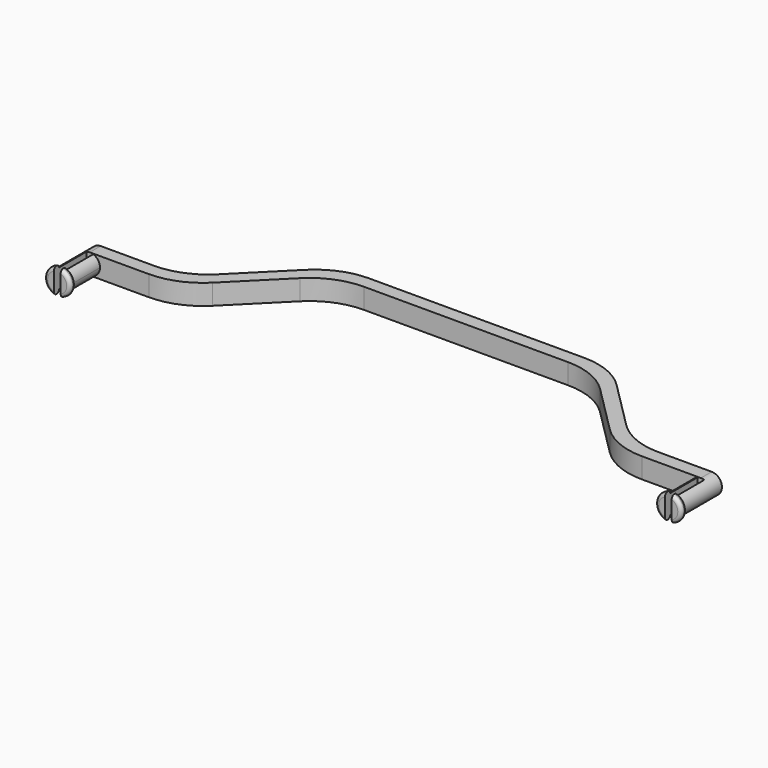
from build123d import *
from build123d import SkipClean  # not in build123d's __all__

# Parameters (mm, degrees)
F1_DEPTH  = 3
F2_R      = 10
F3_R      = 1.5
F4_DEPTH  = 2
F5_DEPTH  = 6
F6_R      = 1.9
F6_R_2    = 1.5
F7_DEPTH  = 1
F9_W      = 1
F9_H      = 10.6840910192
F9_W_2    = 7.2588436306
F9_H_2    = 0.5
F9_W_3    = 6.9682821631
F10_DEPTH = 6


# Not quite as in the source:
# - a fillet or chamfer that OpenCascade refuses, or shapes differently, is made with other operations: its cross-section is extruded or revolved along the edge and cut away or added
# - after a boolean that leaves OpenCascade's solid faulty, fix() repairs it


with BuildPart() as f1:
    # F0 (on Top) → F1 (new body)
    with BuildSketch(Plane.XY):
        Polygon((-45, 2), (-45, 0), (-32.1715728753, 0), (-33, 2), align=None)
        Polygon((-33, 2), (-32.1715728753, 0), (-19.1715728753, 13), (-20, 15), align=None)
        Polygon((-20, 15), (-19.1715728753, 13), (0, 13), (0, 15), align=None)
        Polygon((0, 15), (0, 13), (19.1715728753, 13), (20, 15), align=None)
        Polygon((20, 15), (19.1715728753, 13), (32.1715728753, 0), (33, 2), align=None)
        Polygon((33, 2), (32.1715728753, 0), (45, 0), (45, 2), align=None)
    extrude(amount=F1_DEPTH)

    # F2
    f2_edges = [f1.edges().sort_by_distance(p)[0] for p in [
        (-33, 2, 1.5),
        (-20, 15, 1.5),
        (20, 15, 1.5),
        (33, 2, 1.5),
        (32.171573, 0, 1.5),
        (19.171573, 13, 1.5),
        (-19.171573, 13, 1.5),
        (-32.171573, 0, 1.5),
    ]]
    fillet(f2_edges, radius=F2_R)

    # F3 (on face) → F4 (join, through all)
    with BuildSketch(Plane.XZ):
        with BuildLine():
            Line((-45, 0), (-45, 3))
            ThreePointArc((-45, 3), (-46.5, 1.5), (-45, 0))
        make_face()
        with Locations((45, 1.5)):
            Circle(F3_R)
    extrude(amount=-F4_DEPTH)

    # F3 (on face) → F5 (join)
    with BuildSketch(Plane.XZ):
        with BuildLine():
            Line((-45, 0), (-45, 3))
            ThreePointArc((-45, 3), (-46.5, 1.5), (-45, 0))
        make_face()
        with BuildLine():
            ThreePointArc((-45, 0), (-43.9393398282, 0.4393398282), (-43.5, 1.5))
            ThreePointArc((-43.5, 1.5), (-43.9393398282, 2.5606601718), (-45, 3))
            Line((-45, 3), (-45, 0))
        make_face()
        with Locations((45, 1.5)):
            Circle(F3_R)
    with SkipClean():  # cleaning this boolean's faces spoils the solid; the shape is the same uncleaned
        extrude(amount=F5_DEPTH)

    # F6 (on face) → F7 (join)
    with BuildSketch(Plane.XZ.offset(6)):
        with Locations((-45, 1.5)):
            Circle(F6_R)
        with Locations((-45, 1.5)):
            Circle(F6_R_2, mode=Mode.SUBTRACT)
        with Locations((45, 1.5)):
            Circle(F6_R)
    extrude(amount=-F7_DEPTH)

    add(f1.part.fix(), mode=Mode.REPLACE)

    # F8: fillet of radius 0.5 on 4 edges, made by hand

    # F8_s1 → F8_t2 (revolve, cut)
    with BuildSketch(Plane.XY.offset(1.5)):
        with BuildLine():
            ThreePointArc((-43.1, -5.5), (-43.2464466094, -5.8535533906), (-43.6, -6))
            Line((-43.6, -6), (-43.1, -6))
            Line((-43.1, -6), (-43.1, -5.5))
        make_face()
    revolve(axis=Axis((-45, -6, 1.5), (0, -1, 0)), mode=Mode.SUBTRACT)

    # F8_s3 → F8_t4 (revolve, cut)
    with BuildSketch(Plane.XY.offset(1.5)):
        with BuildLine():
            ThreePointArc((-43.5, -5), (-43.2127016654, -5.1736701825), (-43.1, -5.4898979486))
            Line((-43.1, -5.4898979486), (-43.1, -5))
            Line((-43.1, -5), (-43.5, -5))
        make_face()
    revolve(axis=Axis((-45, -5, 1.5), (0, -1, 0)), mode=Mode.SUBTRACT)

    # F8_s5 → F8_t6 (revolve, cut)
    with BuildSketch(Plane.XY.offset(1.5)):
        with BuildLine():
            ThreePointArc((46.5, -5), (46.7872983346, -5.1736701825), (46.9, -5.4898979486))
            Line((46.9, -5.4898979486), (46.9, -5))
            Line((46.9, -5), (46.5, -5))
        make_face()
    revolve(axis=Axis((45, -5, 1.5), (0, -1, 0)), mode=Mode.SUBTRACT)

    # F8_s7 → F8_t8 (revolve, cut)
    with BuildSketch(Plane.XY.offset(1.5)):
        with BuildLine():
            ThreePointArc((46.9, -5.5), (46.7535533906, -5.8535533906), (46.4, -6))
            Line((46.4, -6), (46.9, -6))
            Line((46.9, -6), (46.9, -5.5))
        make_face()
    revolve(axis=Axis((45, -6, 1.5), (0, -1, 0)), mode=Mode.SUBTRACT)

    # F9 (on face) → F10 (cut, through all)
    with BuildSketch(Plane.XZ.offset(6)):
        with Locations((-45, 1.5)):
            Rectangle(F9_W, F9_H)
        with Locations((-54.3349329382, 3.15)):
            Rectangle(F9_W_2, F9_H_2)
        with Locations((-54.1896522045, -0.15)):
            Rectangle(F9_W_3, F9_H_2)
        with Locations((54.1896522045, -0.15)):
            Rectangle(F9_W_3, F9_H_2)
        with Locations((54.3349329382, 3.15)):
            Rectangle(F9_W_2, F9_H_2)
        with Locations((45, 1.5)):
            Rectangle(F9_W, F9_H)
    extrude(amount=-F10_DEPTH, mode=Mode.SUBTRACT)


solid = f1.part
